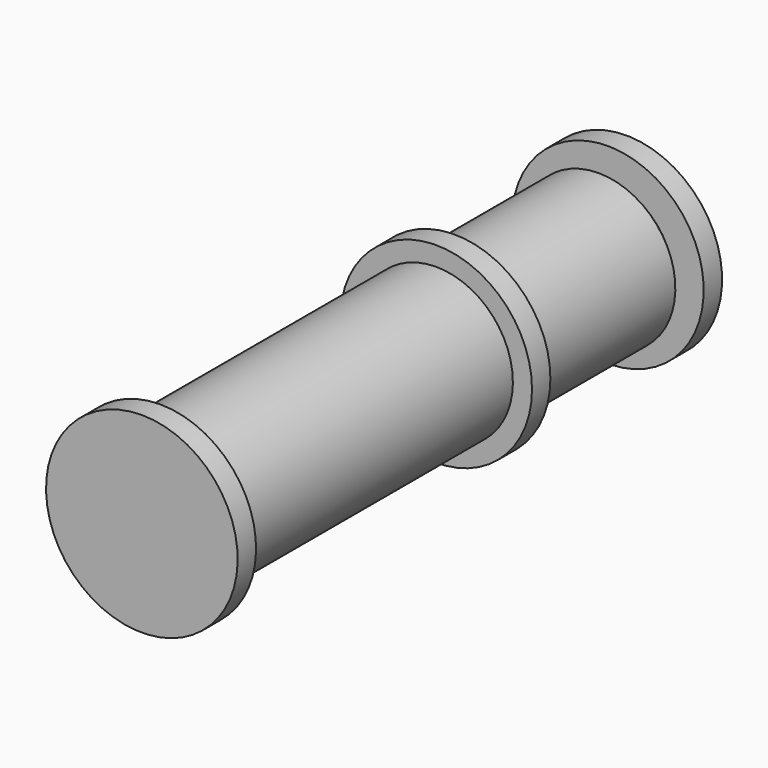
from build123d import *

# Parameters (mm, degrees)
F4_D            = 9
F4_DEPTH        = 6.3
F4_CSINK_D      = 17.92
F4_CSINK_ANGLE  = 90
F4_TIP          = 2.7038727856
F6_D            = 6.8
F6_DEPTH        = 15.75
F6_TIP          = 2.0429261047
F8_R            = 12.5
F9_DEPTH        = 3
F11_D           = 6.8
F11_DEPTH       = 15.75
F11_CSINK_D     = 17.92
F11_CSINK_ANGLE = 90
F11_TIP         = 2.0429261047
F12_SIZE        = 0.5
F14_R           = 12.5
F14_R_2         = 10
F15_DEPTH       = 3


with BuildPart() as f1:
    # F0 (on Right) → F1 (revolve)
    with BuildSketch(Plane.YZ):
        Polygon((-37.5, 12.5), (-37.5, 0), (37.5, 0), (37.5, 10), (-34.5, 10), (-34.5, 12.5), align=None)
    revolve(axis=Axis((0, 0, 0), (0, 1, 0)))

    # F4
    with Locations(Plane(origin=(0, 40.5, 0), x_dir=(-1, 0, 0), z_dir=(0, 1, 0))):
        with Locations((0, 0)):
            CounterSinkHole(F4_D / 2, F4_CSINK_D / 2, depth=F4_DEPTH, counter_sink_angle=F4_CSINK_ANGLE)
            with Locations((0, 0, -(F4_DEPTH + F4_TIP / 2))):  # 118° drill point
                Cone(0, F4_D / 2, F4_TIP, mode=Mode.SUBTRACT)

    # F6
    with Locations(Plane(origin=(0, 37.5, 0), x_dir=(-1, 0, 0), z_dir=(0, 1, 0))):
        with Locations((0, 0)):
            Hole(F6_D / 2, depth=F6_DEPTH)
            with Locations((0, 0, -(F6_DEPTH + F6_TIP / 2))):  # 118° drill point
                Cone(0, F6_D / 2, F6_TIP, mode=Mode.SUBTRACT)

    # F12
    f12_edges = [f1.edges().sort_by_distance(p)[0] for p in [
        (0, 37.5, -10),
    ]]
    chamfer(f12_edges, length=F12_SIZE)


with BuildPart() as f9:
    # F8 (on offset) → F9 (new body)
    with BuildSketch(Plane(origin=(0, 38.5, 0), x_dir=(-1, 0, 0), z_dir=(0, 1, 0))):
        Circle(F8_R)
    extrude(amount=F9_DEPTH)

    # F11
    with Locations(Plane(origin=(0, 41.5, 0), x_dir=(-1, 0, 0), z_dir=(0, 1, 0))):
        with Locations((0, 0)):
            CounterSinkHole(F11_D / 2, F11_CSINK_D / 2, depth=F11_DEPTH, counter_sink_angle=F11_CSINK_ANGLE)
            with Locations((0, 0, -(F11_DEPTH + F11_TIP / 2))):  # 118° drill point
                Cone(0, F11_D / 2, F11_TIP, mode=Mode.SUBTRACT)


with BuildPart() as f15:
    # F14 (on offset) → F15 (new body)
    with BuildSketch(Plane.XZ.offset(-13.5)):
        Circle(F14_R)
        Circle(F14_R_2, mode=Mode.SUBTRACT)
    extrude(amount=F15_DEPTH)


solid = Compound([f1.part, f9.part, f15.part])
